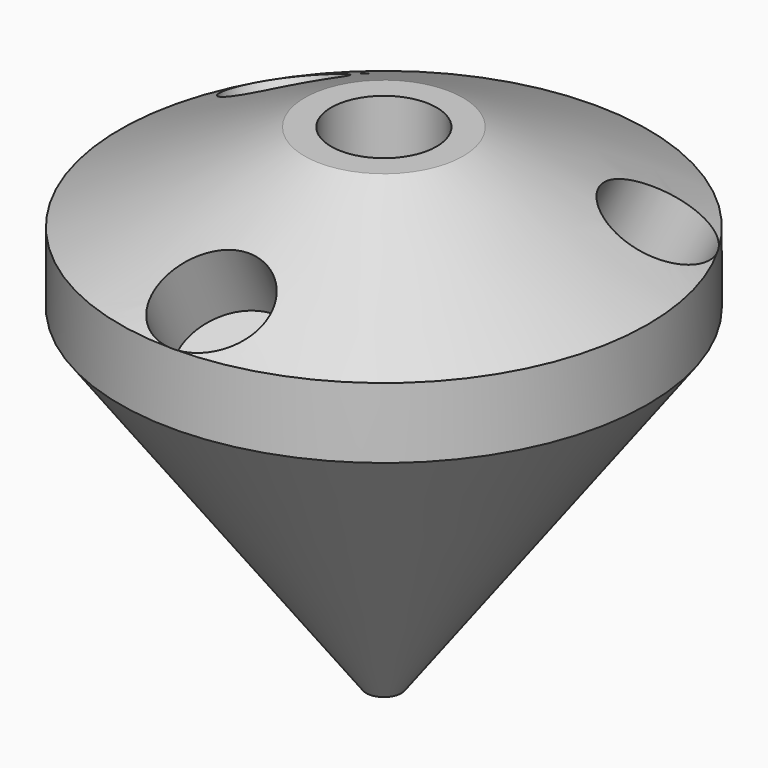
from build123d import *

# Parameters (mm, degrees)
F5_R            = 3
F6_DEPTH        = 4.2
F6_COPIES_COUNT = 3
F8_R            = 3
F9_DEPTH        = 15


# Not quite as in the source:
# - a pattern or mirror of a feature is missing from the dataset's text; its kind, count and spacing are read off the source's solid


with BuildPart() as f2:
    # F0 (on Front) → F2 (revolve)
    with BuildSketch(Plane.XZ):
        Polygon((4.5, 15), (0, 15), (0, -13), (1, -13), (15, 6), (15, 10), align=None)
    revolve(axis=Axis((0, 0, -1.4754105359), (0, 0, -1)))

    # F5 (on line) → F6 (cut)
    with BuildSketch(Plane(origin=(0, -6.6543438078, 13.9741219963), x_dir=(1, 0, 0), z_dir=(0, -0.4299335804, 0.9028605188))):
        with Locations((0, -6.2435719784)):
            Circle(F5_R)
    f6 = extrude(amount=-F6_DEPTH, mode=Mode.SUBTRACT)

    # F6_copies: F6 ×3 about axis
    f6_copies_axis = Axis((0, 0, 0), (0, 0, 1))
    for i in range(1, F6_COPIES_COUNT):
        add(f6.rotate(f6_copies_axis, i * 360 / F6_COPIES_COUNT), mode=Mode.SUBTRACT)

    # F8 (on face) → F9 (cut)
    with BuildSketch(Plane.XY.offset(15)):
        Circle(F8_R)
    extrude(amount=-F9_DEPTH, mode=Mode.SUBTRACT)


solid = f2.part
